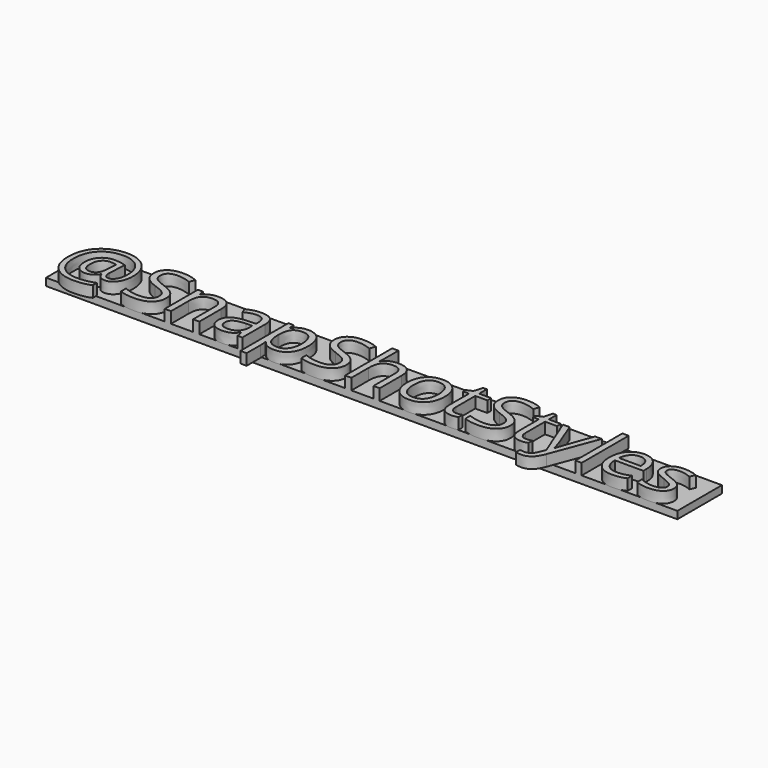
from build123d import *

# Parameters (mm, degrees)
F0_W         = 431.8
F0_H         = 38.1
F1_DEPTH     = 5.08
F2_TEXT_SIZE = 52.9166666667
F3_DEPTH     = 7.62


# Not quite as in the source:
# - Text() gives the source's letters only with a copy of the font that has no kerning and outlines rounded to 1/6400 em; it was checked with that copy


with BuildPart() as f1:
    # F0 (on Top) → F1 (new body)
    with BuildSketch(Plane.XY):
        with Locations((186.6170450181, 3.1541432271)):
            Rectangle(F0_W, F0_H)
    extrude(amount=F1_DEPTH)

    # F2 (on face) → F3 (join)
    with BuildSketch(Plane.XY.offset(5.08)):
        with Locations((-29.2829549819, -15.8958567729)):
            Text('@SnapShotStyles', F2_TEXT_SIZE, font='Open Sans', text_align=(TextAlign.LEFT, TextAlign.BOTTOM))
    extrude(amount=F3_DEPTH)


solid = f1.part
